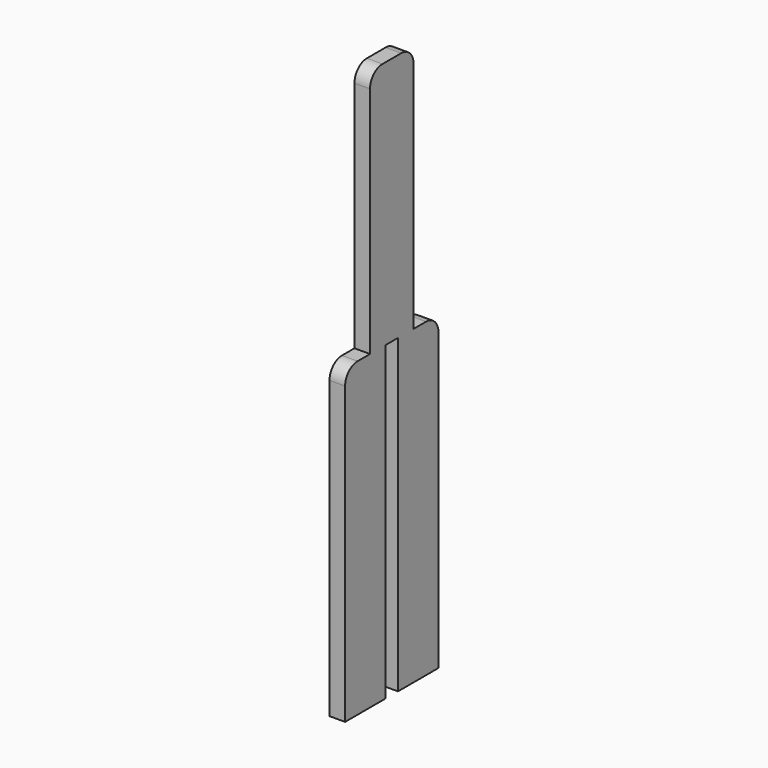
from build123d import *

# Parameters (mm, degrees)
F1_DEPTH = 3.175


# Not quite as in the source:
# - ends of sketch curves that miss each other by under 0.0002 mm in the source are joined


with BuildPart() as f1:
    # F0 (on Right) → F1 (new body, symmetric)
    with BuildSketch(Plane.YZ):
        with BuildLine():
            Line((3.175, -63.5), (23.8125, -63.5))
            Line((23.8125, -63.5), (23.8125, 57.15))
            ThreePointArc((23.8125, 57.15), (21.9533763667, 61.6393796296), (17.4646167058, 63.4999996472))
            Line((17.4646167058, 63.4999996472), (17.4625, 63.5))
            Line((17.4625, 63.5), (11.1139111112, 63.5))
            Line((11.1139111112, 63.5), (11.124494366, 158.7492930333))
            ThreePointArc((11.124494366, 158.7492930333), (9.2648719104, 163.2398771909), (4.7744944052, 165.0999985889))
            Line((4.7744944052, 165.0999985889), (-4.7498, 165.0999985889))
            ThreePointArc((-4.7498, 165.0999985889), (-9.2399280605, 163.2401266494), (-11.0998, 158.7499985889))
            Line((-11.0998, 158.7499985889), (-11.0998, 63.5))
            Line((-11.0998, 63.5), (-17.4498, 63.5))
            Line((-17.4498, 63.5), (-17.4625, 63.5))
            ThreePointArc((-17.4625, 63.5), (-21.9526280605, 61.6401280605), (-23.8125, 57.15))
            Line((-23.8125, 57.15), (-23.8125, -63.5))
            Line((-23.8125, -63.5), (-3.175, -63.5))
            Line((-3.175, -63.5), (-3.175, 63.5))
            Line((-3.175, 63.5), (3.175, 63.5))
            Line((3.175, 63.5), (3.175, -63.5))
        make_face()
    extrude(amount=F1_DEPTH, both=True)


solid = f1.part
